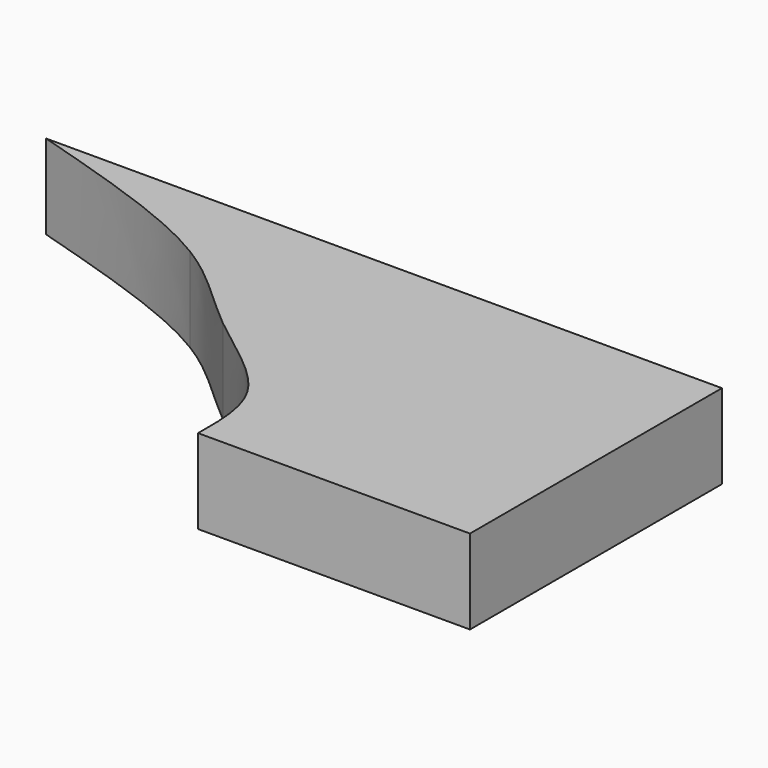
from build123d import *

# Parameters (mm, degrees)
F1_DEPTH = 25.4


with BuildPart() as f1:
    # F0 (on Top) → F1 (new body)
    with BuildSketch(Plane.XY):
        with BuildLine():
            Line((62.1568927622, 331.9272), (203.2, 331.9272))
            Line((203.2, 331.9272), (203.2, 355.6))
            Line((203.2, 355.6), (0, 355.6))
            add(Edge.make_bspline(
                [(62.1568927622, 331.9272), (46.5258539889, 341.4800694919), (23.2629269944, 348.540034746), (0, 355.6)],
                knots=[0.6752877262, 0.6752877262, 0.6752877262, 0.6752877262, 1, 1, 1, 1], degree=3))
        make_face()
        with BuildLine():
            Line((91.0151283785, 308.2544), (203.2, 308.2544))
            Line((203.2, 308.2544), (203.2, 331.9272))
            Line((203.2, 331.9272), (62.1568927622, 331.9272))
            add(Edge.make_bspline(
                [(91.0151283785, 308.2544), (81.293107614, 316.2156971088), (73.8664451152, 324.7709369352), (62.1568927622, 331.9272)],
                knots=[0.4320386737, 0.4320386737, 0.4320386737, 0.4320386737, 0.6752877262, 0.6752877262, 0.6752877262, 0.6752877262], degree=3))
        make_face()
        with BuildLine():
            Line((117.3283786334, 284.5816), (203.2, 284.5816))
            Line((203.2, 284.5816), (203.2, 308.2544))
            Line((203.2, 308.2544), (91.0151283785, 308.2544))
            add(Edge.make_bspline(
                [(117.3283786334, 284.5816), (112.1261985969, 293.312325694), (100.4823531117, 300.5017536394), (91.0151283785, 308.2544)],
                knots=[0.1951647253, 0.1951647253, 0.1951647253, 0.1951647253, 0.4320386737, 0.4320386737, 0.4320386737, 0.4320386737], degree=3))
        make_face()
        with BuildLine():
            Line((121.441156018, 260.9088), (203.2, 260.9088))
            Line((203.2, 260.9088), (203.2, 284.5816))
            Line((203.2, 284.5816), (117.3283786334, 284.5816))
            add(Edge.make_bspline(
                [(121.441156018, 260.9088), (121.5278523804, 269.1484986902), (121.6145487428, 277.3881973804), (117.3283786334, 284.5816)],
                knots=[0, 0, 0, 0, 0.1951647253, 0.1951647253, 0.1951647253, 0.1951647253], degree=3))
        make_face()
    extrude(amount=F1_DEPTH)


solid = f1.part
